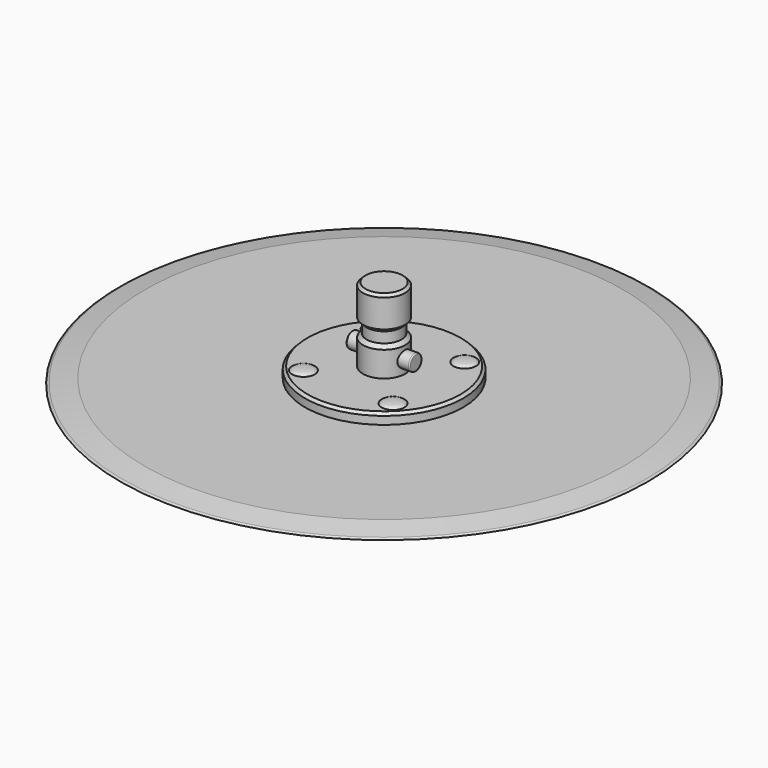
from build123d import *

# Parameters (mm, degrees)
F0_R      = 50
F0_R_2    = 1.5
F0_R_3    = 9
F1_DEPTH  = 1
F6_SIZE   = 0.5
F7_SIZE   = 0.69999
F8_R      = 15
F9_DEPTH  = 1.1
F12_W     = 1.5
F12_H     = 3
F12_H_2   = 1.1
F14_COUNT = 4
F15_R     = 1.5
F16_DEPTH = 6
F17_R     = 0.2


# Not quite as in the source:
# - a fillet or chamfer is up to 0.001 mm smaller than in the source, because OpenCascade refuses the exact size


with BuildPart() as f1:
    # F0 (on Top) → F1 (new body)
    with BuildSketch(Plane.XY):
        Circle(F0_R)
        with Locations((-8.4852813742, -8.4852813742)):
            Circle(F0_R_2, mode=Mode.SUBTRACT)
        with Locations((8.4852813742, -8.4852813742)):
            Circle(F0_R_2, mode=Mode.SUBTRACT)
        with Locations((-8.4852813742, 8.4852813742)):
            Circle(F0_R_2, mode=Mode.SUBTRACT)
        Circle(F0_R_3, mode=Mode.SUBTRACT)
        with Locations((8.4852813742, 8.4852813742)):
            Circle(F0_R_2, mode=Mode.SUBTRACT)
    extrude(amount=F1_DEPTH)

    # F2 (on Front) → F3 (revolve, cut)
    with BuildSketch(Plane.XZ):
        Polygon((49.5669872981, 0.25), (50, 0), (52.7446980246, 3.1410633654), (39.3594096073, 2.0498713546), align=None)
    revolve(axis=Axis((0, 0, -4.0544420481), (0, 0, -1)), mode=Mode.SUBTRACT)


with BuildPart() as f5:
    # F4 (on Front) → F5 (revolve)
    with BuildSketch(Plane.XZ):
        Polygon((4, 17), (0, 17), (0, 0), (9, 0), (9, 1), (15, 1), (15, 3), (4, 3), (4, 8.5), (3.3, 8.5), (3.3, 10.5), (4, 10.5), align=None)
    revolve(axis=Axis((0, 0, -7.3282243684), (0, 0, -1)))

    # F6
    f6_edges = [f5.edges().sort_by_distance(p)[0] for p in [
        (-4, 0, 17),
        (-15, 0, 3),
    ]]
    chamfer(f6_edges, length=F6_SIZE)

    # F7 (size 0.7 in the source; OpenCascade refuses exactly that, so slightly less here)
    f7_edges = [f5.edges().sort_by_distance(p)[0] for p in [
        (-4, 0, 8.5),
        (-4, 0, 10.5),
    ]]
    chamfer(f7_edges, length=F7_SIZE)

    # F15 (on Right) → F16 (join, symmetric)
    with BuildSketch(Plane.YZ):
        with Locations((0, 5.5)):
            Circle(F15_R)
    extrude(amount=F16_DEPTH, both=True)

    # F17
    f17_edges = [f5.edges().sort_by_distance(p)[0] for p in [
        (-6, -1.5, 5.5),
        (6, -1.5, 5.5),
    ]]
    fillet(f17_edges, radius=F17_R)


with BuildPart() as f9:
    # F8 (on face) → F9 (new body)
    with BuildSketch(Plane(origin=(0, 0, 0), x_dir=(1, 0, 0), z_dir=(0, 0, -1))):
        Circle(F8_R)
    extrude(amount=F9_DEPTH)


with BuildPart() as f13:
    # F12 (on line) → F13 (revolve)
    with BuildSketch(Plane(origin=(0, 0, 0), x_dir=(-0.7071067812, -0.7071067812, 0), z_dir=(-0.7071067812, 0.7071067812, 0))):
        with BuildLine():
            Line((-14.1390450299, 3), (-13.5, 3))
            Line((-13.5, 3), (-12, 3))
            Line((-12, 3), (-12, 3.4789917991))
            add(Edge.make_bspline(
                [(-14.1390450299, 3), (-13.9814806506, 3.1268322923), (-13.6449454738, 3.3977280881), (-12.8337925749, 3.4748752832), (-12.2812192629, 3.4776033919), (-12, 3.4789917991)],
                knots=[0, 0, 0, 0, 0.3018402139, 0.6446879063, 1, 1, 1, 1], degree=3))
        make_face()
        with Locations((-12.75, 1.5)):
            Rectangle(F12_W, F12_H)
        Polygon((-12, -1.1), (-13.5, -1.1), (-14.9, -1.1), (-14.9, -1.6), (-12, -1.6), align=None)
        with Locations((-12.75, -0.55)):
            Rectangle(F12_W, F12_H_2)
    revolve(axis=Axis((8.4852813742, 8.4852813742, -0.2961338032), (0, 0, -1)))


with BuildPart() as f14_1:
    # F14: instance of F13
    add(f13.part.rotate(Axis((0, 0, 20.5511674285), (0, 0, 1)), 1 * 360 / F14_COUNT))


with BuildPart() as f14_2:
    # F14: instance of F13
    add(f13.part.rotate(Axis((0, 0, 20.5511674285), (0, 0, 1)), 2 * 360 / F14_COUNT))


with BuildPart() as f14_3:
    # F14: instance of F13
    add(f13.part.rotate(Axis((0, 0, 20.5511674285), (0, 0, 1)), 3 * 360 / F14_COUNT))


solid = Compound([f1.part, f5.part, f9.part, f13.part, f14_1.part, f14_2.part, f14_3.part])
